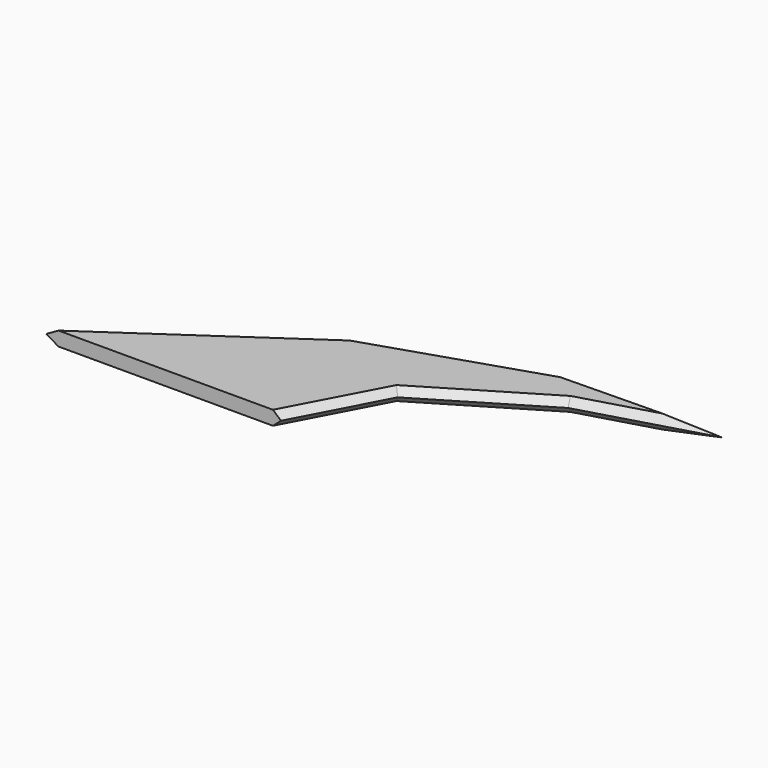
from build123d import *

# Parameters (mm, degrees)
F1_DEPTH = 3
F2_SIZE  = 1.49999


# Not quite as in the source:
# - a fillet or chamfer is up to 0.001 mm smaller than in the source, because OpenCascade refuses the exact size


with BuildPart() as f1:
    # F0 (on Top) → F1 (new body)
    with BuildSketch(Plane.XY):
        Polygon((-50, 0), (0, 0), (9.9, 18.7), (34.4, 33.4), (61, 41.1), (28, 40.5), (-8, 28.8), align=None)
    extrude(amount=F1_DEPTH)

    # F2 (size 1.5 in the source; OpenCascade refuses exactly that, so slightly less here)
    f2_edges = [f1.edges().sort_by_distance(p)[0] for p in [
        (-29, 14.4, 3),
        (10, 34.65, 3),
        (10, 34.65, 0),
        (-29, 14.4, 0),
        (44.5, 40.8, 0),
        (44.5, 40.8, 3),
        (47.7, 37.25, 3),
        (47.7, 37.25, 0),
        (22.15, 26.05, 3),
        (22.15, 26.05, 0),
        (4.95, 9.35, 3),
        (4.95, 9.35, 0),
    ]]
    chamfer(f2_edges, length=F2_SIZE)


solid = f1.part
